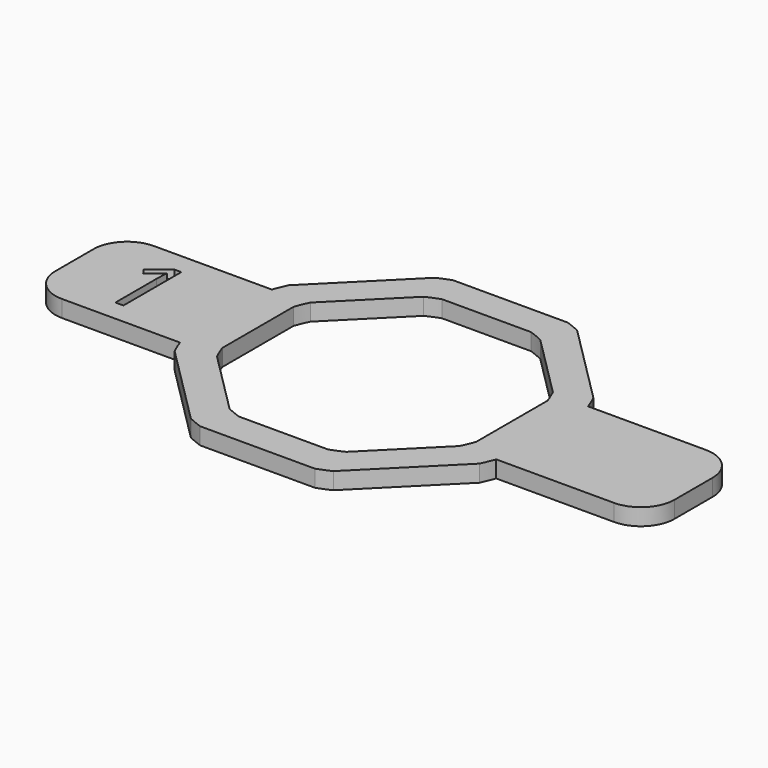
from build123d import *

# Parameters (mm, degrees)
F1_DEPTH     = 1.27
F0_TEXT_SIZE = 7.6509245749
F2_DEPTH     = 0.635


# Not quite as in the source:
# - Text() gives the source's letters only with a copy of the font that has no kerning and outlines rounded to 1/6400 em; it was checked with that copy


with BuildPart() as f1:
    # F0 (on Top) → F1 (new body)
    with BuildSketch(Plane.XY):
        with BuildLine():
            Line((-5.377606881, 11.5052746266), (-11.5052746266, 5.377606881))
            ThreePointArc((-11.5052746266, 5.377606881), (-11.7332700629, 4.860079591), (-11.938, 4.3329154157))
            Line((-11.938, 4.3329154157), (-11.938, -4.3329154157))
            ThreePointArc((-11.938, -4.3329154157), (-11.7332700629, -4.860079591), (-11.5052746266, -5.377606881))
            Line((-11.5052746266, -5.377606881), (-5.377606881, -11.5052746266))
            ThreePointArc((-5.377606881, -11.5052746266), (-4.860079591, -11.7332700629), (-4.3329154157, -11.938))
            Line((-4.3329154157, -11.938), (4.3329154157, -11.938))
            ThreePointArc((4.3329154157, -11.938), (4.860079591, -11.7332700629), (5.377606881, -11.5052746266))
            Line((5.377606881, -11.5052746266), (11.5052746266, -5.377606881))
            ThreePointArc((11.5052746266, -5.377606881), (11.7332700629, -4.860079591), (11.938, -4.3329154157))
            Line((11.938, -4.3329154157), (11.938, 4.3329154157))
            ThreePointArc((11.938, 4.3329154157), (11.7332700629, 4.860079591), (11.5052746266, 5.377606881))
            Line((11.5052746266, 5.377606881), (5.377606881, 11.5052746266))
            ThreePointArc((5.377606881, 11.5052746266), (4.860079591, 11.7332700629), (4.3329154157, 11.938))
            Line((4.3329154157, 11.938), (-4.3329154157, 11.938))
            ThreePointArc((-4.3329154157, 11.938), (-4.860079591, 11.7332700629), (-5.377606881, 11.5052746266))
        make_face()
        with BuildLine():
            ThreePointArc((9.185876282, 4.4536252577), (9.4168708354, 3.9371236846), (9.6187547851, 3.4085641046))
            Line((9.6187547851, 3.4085641046), (9.6187547851, -3.3104440811))
            ThreePointArc((9.6187547851, -3.3104440811), (9.4168708354, -3.8390036611), (9.185876282, -4.3555052341))
            Line((9.185876282, -4.3555052341), (4.434820031, -9.1065614851))
            ThreePointArc((4.434820031, -9.1065614851), (3.9183184579, -9.3375560385), (3.389758878, -9.5394399882))
            Line((3.389758878, -9.5394399882), (-3.3292493078, -9.5394399882))
            ThreePointArc((-3.3292493078, -9.5394399882), (-3.8578088877, -9.3375560385), (-4.3743104608, -9.1065614851))
            Line((-4.3743104608, -9.1065614851), (-9.1253667118, -4.3555052341))
            ThreePointArc((-9.1253667118, -4.3555052341), (-9.3563612652, -3.8390036611), (-9.5582452149, -3.3104440811))
            Line((-9.5582452149, -3.3104440811), (-9.5582452149, 3.4085641046))
            ThreePointArc((-9.5582452149, 3.4085641046), (-9.3563612652, 3.9371236846), (-9.1253667118, 4.4536252577))
            Line((-9.1253667118, 4.4536252577), (-4.3743104608, 9.2046815087))
            ThreePointArc((-4.3743104608, 9.2046815087), (-3.8578088877, 9.4356760621), (-3.3292493078, 9.6375600118))
            Line((-3.3292493078, 9.6375600118), (3.389758878, 9.6375600118))
            ThreePointArc((3.389758878, 9.6375600118), (3.9183184579, 9.4356760621), (4.434820031, 9.2046815087))
            Line((4.434820031, 9.2046815087), (9.185876282, 4.4536252577))
        make_face(mode=Mode.SUBTRACT)
        with BuildLine():
            Line((-11.938, -4.3329154157), (-11.938, 4.3329154157))
            Line((-11.938, 4.3329154157), (-20.828, 4.3329154157))
            ThreePointArc((-20.828, 4.3329154157), (-22.6240512242, 3.58896664), (-23.368, 1.7929154157))
            Line((-23.368, 1.7929154157), (-23.368, -1.7929154157))
            ThreePointArc((-23.368, -1.7929154157), (-22.6240512242, -3.58896664), (-20.828, -4.3329154157))
            Line((-20.828, -4.3329154157), (-11.938, -4.3329154157))
        make_face()
        with BuildLine():
            Line((-17.4945113016, 2.7395427473), (-17.4945113016, -2.7225001249))
            Line((-17.4945113016, -2.7225001249), (-18.0994125258, -2.7225001249))
            Line((-18.0994125258, -2.7225001249), (-18.0994125258, 1.1699077525))
            add(Edge.make_bspline(
                [(-18.0994125258, 1.1699077525), (-18.0994125258, 1.6564587372), (-18.0695261017, 2.0892141585)],
                knots=[0, 0, 0, 1, 1, 1], degree=2))
            add(Edge.make_bspline(
                [(-18.0695261017, 2.0892141585), (-18.1472308044, 2.0103139988), (-18.244660547, 1.9248388258)],
                knots=[0, 0, 0, 1, 1, 1], degree=2))
            add(Edge.make_bspline(
                [(-18.244660547, 1.9248388258), (-18.3420902896, 1.8393636528), (-19.1334828003, 1.1962078058)],
                knots=[0, 0, 0, 1, 1, 1], degree=2))
            Line((-19.1334828003, 1.1962078058), (-19.4622334657, 1.6217904852))
            Line((-19.4622334657, 1.6217904852), (-18.0169259952, 2.7395427473))
            Line((-18.0169259952, 2.7395427473), (-17.4945113016, 2.7395427473))
        make_face(mode=Mode.SUBTRACT)
        with BuildLine():
            Line((20.828, 4.3329154157), (11.938, 4.3329154157))
            Line((11.938, 4.3329154157), (11.938, -4.3329154157))
            Line((11.938, -4.3329154157), (20.828, -4.3329154157))
            ThreePointArc((20.828, -4.3329154157), (22.6240512242, -3.58896664), (23.368, -1.7929154157))
            Line((23.368, -1.7929154157), (23.368, 1.7929154157))
            ThreePointArc((23.368, 1.7929154157), (22.6240512242, 3.58896664), (20.828, 4.3329154157))
        make_face()
    extrude(amount=F1_DEPTH)

    # F0 (on Top) → F2 (join)
    with BuildSketch(Plane.XY):
        with Locations((-20.165162161, -2.7225001249)):
            Text('1', F0_TEXT_SIZE, font='Open Sans', text_align=(TextAlign.LEFT, TextAlign.BOTTOM))
    extrude(amount=F2_DEPTH)


solid = f1.part
